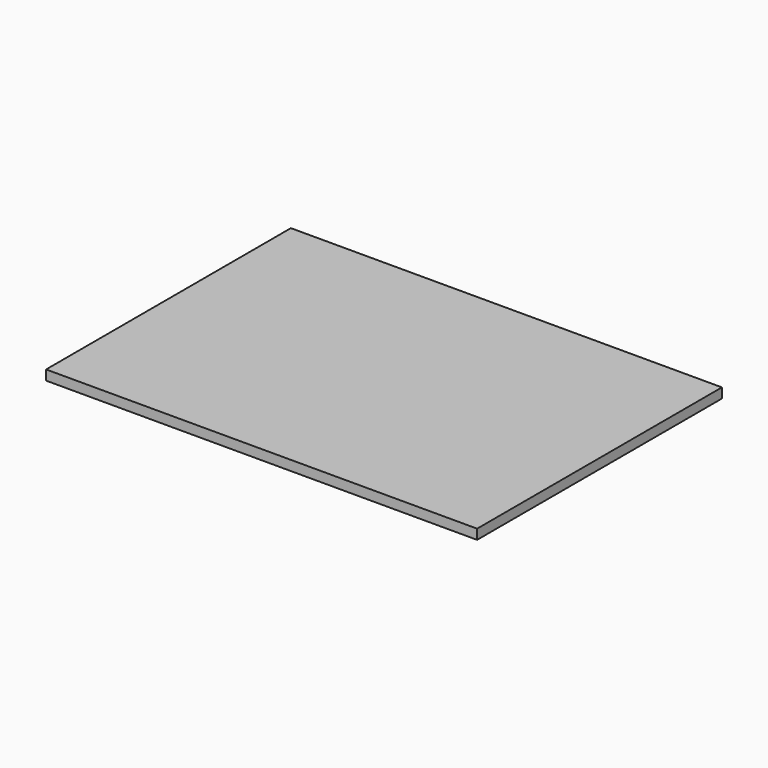
from build123d import *

# Parameters (mm, degrees)
F0_W      = 500
F0_H      = 500
F1_DEPTH  = 12
F2_W      = 500
F2_H      = 50
F3_DEPTH  = 6
F6_DEPTH  = 6
F14_DEPTH = 6
F15_R     = 19.99999
F19_DEPTH = 6
F22_DEPTH = 12
F25_DEPTH = 6
F27_W     = 12
F27_H     = 320
F28_DEPTH = 44
F31_W     = 196
F31_H     = 12
F32_DEPTH = 44
F37_DEPTH = 3
F43_DEPTH = 12


# Not quite as in the source:
# - a fillet or chamfer is up to 0.001 mm smaller than in the source, because OpenCascade refuses the exact size


with BuildPart() as f1:
    # F0 (on Top) → F1 (new body)
    with BuildSketch(Plane.XY):
        Rectangle(F0_W, F0_H)
    extrude(amount=F1_DEPTH)


with BuildPart() as f3:
    # F2 (on Right) → F3 (new body, symmetric)
    with BuildSketch(Plane.YZ):
        Rectangle(F2_W, F2_H)
    extrude(amount=F3_DEPTH, both=True)


with BuildPart() as f3_1:
    # F4: moved
    add(f3.part.moved(Location((0, 0, -25))))


with BuildPart() as f6:
    # F5 (on Front) → F6 (new body, symmetric)
    with BuildSketch(Plane.XZ):
        Polygon((-250, -25), (250, -25), (250, 25), (6, 25), (6, 0), (-6, 0), (-6, 25), (-250, 25), align=None)
    extrude(amount=F6_DEPTH, both=True)


with BuildPart() as f6_1:
    # F7: moved
    add(f6.part.moved(Location((0, 80, -25))))


with BuildPart() as f8_1:
    # F8: copy of F6
    add(f6_1.part)


with BuildPart() as f3_2:
    add(f3_1.part)

    # F10: cut F6
    add(f6_1.part, mode=Mode.SUBTRACT)


with BuildPart() as f11_1:
    # F11: copy of F6
    add(f6_1.part.moved(Location((0, 164, 0))))


with BuildPart() as f3_3:
    add(f3_2.part)

    # F12: cut F11_1
    add(f11_1.part, mode=Mode.SUBTRACT)


with BuildPart() as f14:
    # F13 (on Right) → F14 (new body, symmetric)
    with BuildSketch(Plane.YZ):
        Polygon((250, -50), (250, 0), (250, 452), (70, 452), (-110, 452), (-250, 100), (-250, -50), align=None)
        Polygon((0, 412), (70, 412), (140, 412), (140, 372), (0, 372), align=None, mode=Mode.SUBTRACT)
    extrude(amount=F14_DEPTH, both=True)

    # F15 (radius 20 in the source; OpenCascade refuses exactly that, so slightly less here)
    f15_edges = [f14.edges().sort_by_distance(p)[0] for p in [
        (0, 140, 372),
        (0, 140, 412),
        (0, 0, 412),
        (0, 0, 372),
    ]]
    fillet(f15_edges, radius=F15_R)


with BuildPart() as f14_1:
    # F16: moved
    add(f14.part.moved(Location((-256, 0, 0))))


with BuildPart() as f17_1:
    # F17: copy of F14
    add(f14_1.part.moved(Location((512, 0, 0))))


with BuildPart() as f19:
    # F18 (on Front) → F19 (new body, symmetric)
    with BuildSketch(Plane.XZ):
        Polygon((-262, 452), (-262, 0), (-262, -50), (262, -50), (262, 452), align=None)
    extrude(amount=F19_DEPTH, both=True)


with BuildPart() as f19_1:
    # F20: moved
    add(f19.part.moved(Location((0, 256, 0))))


with BuildPart() as f22:
    # F21 (on face) → F22 (new body)
    with BuildSketch(Plane.XY.offset(12)):
        Polygon((262, 262), (0, 262), (-262, 262), (-262, -110), (262, -110), align=None)
    extrude(amount=F22_DEPTH)


with BuildPart() as f22_1:
    # F23: moved
    add(f22.part.moved(Location((0, 0, 440))))


with BuildPart() as f25:
    # F24 (on Front) → F25 (new body, symmetric)
    with BuildSketch(Plane.XZ):
        Polygon((-250, 12), (0, 12), (250, 12), (250, 100), (-250, 100), align=None)
    extrude(amount=F25_DEPTH, both=True)


with BuildPart() as f25_1:
    # F26: moved
    add(f25.part.moved(Location((0, -244, 0))))


with BuildPart() as f28:
    # F27 (on Top) → F28 (new body)
    with BuildSketch(Plane.XY):
        with Locations((-24, -90)):
            Rectangle(F27_W, F27_H)
    extrude(amount=F28_DEPTH)


with BuildPart() as f28_1:
    # F29: moved
    add(f28.part.moved(Location((0, 0, -48))))


with BuildPart() as f30_1:
    # F30: copy of F28
    add(f28_1.part.moved(Location((-208, 0, 0))))


with BuildPart() as f32:
    # F31 (on Top) → F32 (new body)
    with BuildSketch(Plane.XY):
        with Locations((-128, -244)):
            Rectangle(F31_W, F31_H)
    extrude(amount=-F32_DEPTH)


with BuildPart() as f32_1:
    # F33: moved
    add(f32.part.moved(Location((0, 0, -4))))


with BuildPart() as f34_1:
    # F34: copy of F32
    add(f32_1.part.moved(Location((0, 308, 0))))


with BuildPart() as f35_1:
    # F35: copy of F32
    add(f32_1.part.moved(Location((256, 0, 0))))


with BuildPart() as f35_2:
    # F35: copy of F30_1
    add(f30_1.part.moved(Location((256, 0, 0))))


with BuildPart() as f35_3:
    # F35: copy of F28
    add(f28_1.part.moved(Location((256, 0, 0))))


with BuildPart() as f35_4:
    # F35: copy of F34_1
    add(f34_1.part.moved(Location((256, 0, 0))))


with BuildPart() as f37:
    # F36 (on Top) → F37 (new body)
    with BuildSketch(Plane.XY):
        Polygon((-24, -244), (-24, 0), (-24, 64), (-232, 64), (-232, -244), align=None)
    extrude(amount=F37_DEPTH)


with BuildPart() as f37_1:
    # F38: moved
    add(f37.part.moved(Location((0, 0, -44))))


with BuildPart() as f39_1:
    # F39: copy of F37
    add(f37_1.part.moved(Location((256, 0, 0))))


with BuildPart() as f30_1_1:
    add(f30_1.part)

    # F40: cut F37
    add(f37_1.part, mode=Mode.SUBTRACT)


with BuildPart() as f32_2:
    add(f32_1.part)

    # F40: cut F37
    add(f37_1.part, mode=Mode.SUBTRACT)


with BuildPart() as f28_2:
    add(f28_1.part)

    # F40: cut F37
    add(f37_1.part, mode=Mode.SUBTRACT)


with BuildPart() as f34_1_1:
    add(f34_1.part)

    # F40: cut F37
    add(f37_1.part, mode=Mode.SUBTRACT)


with BuildPart() as f35_1_1:
    add(f35_1.part)

    # F41: cut F39_1
    add(f39_1.part, mode=Mode.SUBTRACT)


with BuildPart() as f35_3_1:
    add(f35_3.part)

    # F41: cut F39_1
    add(f39_1.part, mode=Mode.SUBTRACT)


with BuildPart() as f35_4_1:
    add(f35_4.part)

    # F41: cut F39_1
    add(f39_1.part, mode=Mode.SUBTRACT)


with BuildPart() as f35_2_1:
    add(f35_2.part)

    # F41: cut F39_1
    add(f39_1.part, mode=Mode.SUBTRACT)


with BuildPart() as f43:
    # F42 (on Front) → F43 (new body)
    with BuildSketch(Plane.XZ):
        Polygon((0, 12), (0, 0), (0, -50), (262, -50), (262, 12), align=None)
    extrude(amount=F43_DEPTH)


with BuildPart() as f43_1:
    # F44: moved
    add(f43.part.moved(Location((0, -250, 0))))


with BuildPart() as f45_1:
    # F45: copy of F43
    add(f43_1.part.moved(Location((-262, 0, 0))))


solid = f22_1.part
